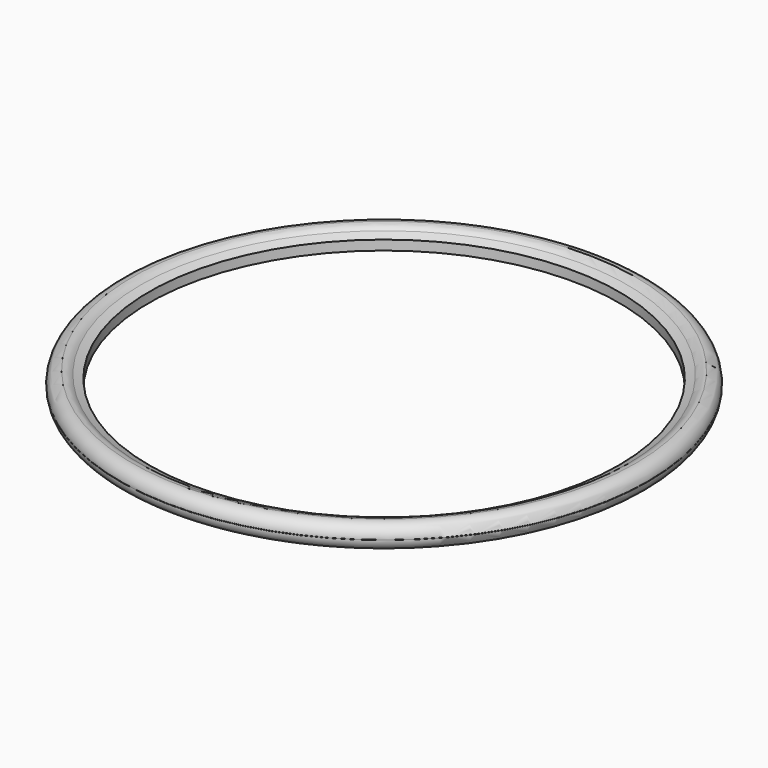
from build123d import *


# Not quite as in the source:
# - a feature names something its author has since deleted; it is built from what else it names


with BuildPart() as f1:
    # F0 (on Front) → F1 (revolve)
    with BuildSketch(Plane.XZ):
        with BuildLine():
            Line((628.65, 0), (615.95, 0))
            Line((615.95, 0), (615.95, -12.7))
            Line((615.95, -12.7), (637.4086206897, -21.8965517241))
            ThreePointArc((637.4086206897, -21.8965517241), (630.9208650644, -11.7916539742), (628.65, 0))
        make_face()
        with BuildLine():
            Line((615.95, 12.7), (615.95, 0))
            Line((615.95, 0), (628.65, 0))
            ThreePointArc((628.65, 0), (630.9208650644, 11.7916539742), (637.4086206897, 21.8965517241))
            Line((637.4086206897, 21.8965517241), (615.95, 12.7))
        make_face()
        with BuildLine():
            ThreePointArc((637.4086206897, 21.8965517241), (630.9208650644, 11.7916539742), (628.65, 0))
            ThreePointArc((628.65, 0), (630.9208650644, -11.7916539742), (637.4086206897, -21.8965517241))
            Line((637.4086206897, -21.8965517241), (660.4, -31.75))
            ThreePointArc((660.4, -31.75), (682.7606574143, -22.5402639736), (692.1489839837, -0.254))
            Line((692.1489839837, -0.254), (689.61, -0.254))
            Line((689.61, -0.254), (689.61, 0))
            Line((689.61, 0), (689.61, 0.254))
            Line((689.61, 0.254), (692.1489839837, 0.254))
            ThreePointArc((692.1489839837, 0.254), (682.7606574143, 22.5402639736), (660.4, 31.75))
            Line((660.4, 31.75), (637.4086206897, 21.8965517241))
        make_face()
        with BuildLine():
            ThreePointArc((660.4, 31.75), (647.8930622701, 29.1828547031), (637.4086206897, 21.8965517241))
            Line((637.4086206897, 21.8965517241), (660.4, 31.75))
        make_face()
        with BuildLine():
            Line((660.4, -31.75), (637.4086206897, -21.8965517241))
            ThreePointArc((637.4086206897, -21.8965517241), (647.8930622701, -29.1828547031), (660.4, -31.75))
        make_face()
    revolve(axis=Axis((0, 0, 41.6052), (0, 0, 1)))


solid = f1.part
